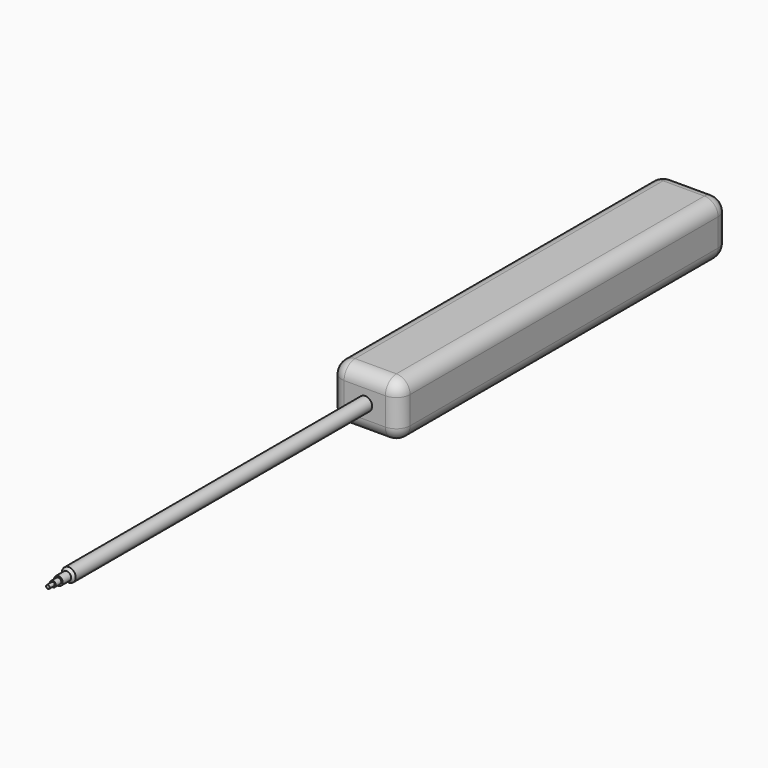
from build123d import *

# Parameters (mm, degrees)
F0_W         = 25.4
F0_H         = 20.32
F1_DEPTH     = 127
F2_R         = 5.08
F3_R         = 5.08
F4_R         = 5.08
F5_DEPTH     = 25.4
F6_R         = 2.54
F7_DEPTH     = 139.192
F8_R         = 5.08
F9_R         = 1.6125595219
F10_DEPTH    = 2.54
F11_R        = 1.0795
F12_DEPTH    = 2.54
F13_R        = 0.680816043
F14_DEPTH    = 2.286
F15_S5_R     = 1.6125595219
F15_T6_DEPTH = 5
F16_R        = 5.1312830473
F17_DEPTH    = 2.286
F18_W        = 15.1486136019
F18_H        = 8.2696229219
F19_DEPTH    = 0.00254


# Not quite as in the source:
# - a fillet or chamfer that OpenCascade refuses, or shapes differently, is made with other operations: its cross-section is extruded or revolved along the edge and cut away or added


with BuildPart() as f1:
    # F0 (on Front) → F1 (new body)
    with BuildSketch(Plane.XZ):
        with Locations((-0.1826275468, -0.0669072086)):
            Rectangle(F0_W, F0_H)
    extrude(amount=F1_DEPTH)

    # F2
    f2_edges = [f1.edges().sort_by_distance(p)[0] for p in [
        (12.517372, -63.5, 10.093093),
        (12.517372, -63.5, -10.226907),
    ]]
    fillet(f2_edges, radius=F2_R)

    # F3
    f3_edges = [f1.edges().sort_by_distance(p)[0] for p in [
        (-12.882628, -63.5, -10.226907),
    ]]
    fillet(f3_edges, radius=F3_R)

    # F4
    f4_edges = [f1.edges().sort_by_distance(p)[0] for p in [
        (-12.882628, -63.5, 10.093093),
        (-12.882628, 0, 2.473093),
    ]]
    fillet(f4_edges, radius=F4_R)

    # F5 (add): a face of the model
    f5_faces = [f1.faces().sort_by_distance(p)[0] for p in [
        (-0.1826275468, -127, -0.0669072086),
    ]]
    extrude(f5_faces, amount=F5_DEPTH)

    # F6 (on face) → F7 (join)
    with BuildSketch(Plane.XZ.offset(152.4)):
        Circle(F6_R)
    extrude(amount=F7_DEPTH)

    # F8
    f8_edges = [f1.edges().sort_by_distance(p)[0] for p in [
        (-0.182628, -152.4, 10.093093),
        (-0.182628, -152.4, -10.226907),
        (12.517372, -152.4, -0.066907),
        (-12.882628, -152.4, -0.066907),
    ]]
    fillet(f8_edges, radius=F8_R)

    # F9 (on face) → F10 (join)
    with BuildSketch(Plane.XZ.offset(291.592)):
        Circle(F9_R)
    extrude(amount=F10_DEPTH)

    # F11 (on face) → F12 (join)
    with BuildSketch(Plane.XZ.offset(294.132)):
        Circle(F11_R)
    extrude(amount=F12_DEPTH)

    # F13 (on face) → F14 (join)
    with BuildSketch(Plane.XZ.offset(296.672)):
        Circle(F13_R)
    extrude(amount=F14_DEPTH)

    # F15: chamfer of 2.286 on 1 edges, made by hand


with BuildPart() as f15_tool2:
    # F15_s3 → F15_t4 (revolve)
    with BuildSketch(Plane.XY):
        Polygon((2.54, -289.306), (0.254, -291.592), (2.54, -291.592), align=None)
    revolve(axis=Axis((0, -291.592, 0), (0, -1, 0)))

    # F15_s5 → F15_t6 (cut, symmetric)
    with BuildSketch(Plane.XZ.offset(290.4)):
        Circle(F15_S5_R)
    extrude(amount=F15_T6_DEPTH, both=True, mode=Mode.SUBTRACT)


with BuildPart() as f1_1:
    add(f1.part)

    # F15_t1: cut F15_tool2
    add(f15_tool2.part, mode=Mode.SUBTRACT)

    # F16 (on face) → F17 (cut)
    with BuildSketch(Plane(origin=(0, 0, -10.2269072086), x_dir=(1, 0, 0), z_dir=(0, 0, -1))):
        with Locations((0, 15.0263812393)):
            Circle(F16_R)
    extrude(amount=-F17_DEPTH, mode=Mode.SUBTRACT)

    # F18 (on face) → F19 (join)
    with BuildSketch(Plane(origin=(0, 0, -10.2269072086), x_dir=(1, 0, 0), z_dir=(0, 0, -1))):
        with Locations((0.0473735854, 139.4127830863)):
            Rectangle(F18_W, F18_H)
    extrude(amount=F19_DEPTH)


solid = f1_1.part
